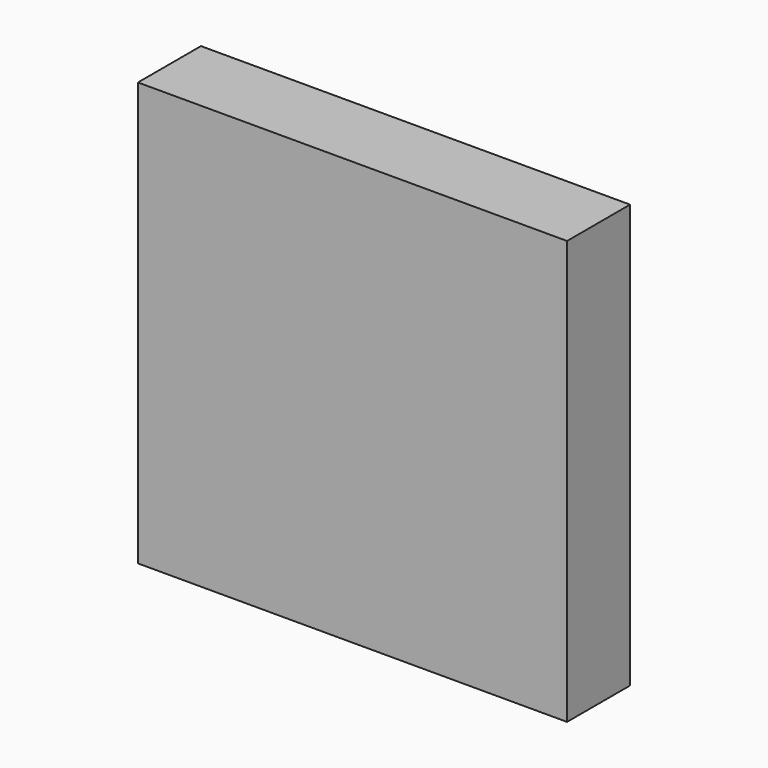
from build123d import *

# Parameters (mm, degrees)
F0_W     = 138.4008337424
F0_H     = 136.5577280521
F1_DEPTH = 25.4


# Not quite as in the source:
# - the program builds the solid bodies; features that only make, move or delete a surface that nothing else refers to are left out


with BuildPart() as f1:
    # F0 (on Front) → F1 (new body)
    with BuildSketch(Plane.XZ):
        Rectangle(F0_W, F0_H)
    extrude(amount=F1_DEPTH)


solid = f1.part
